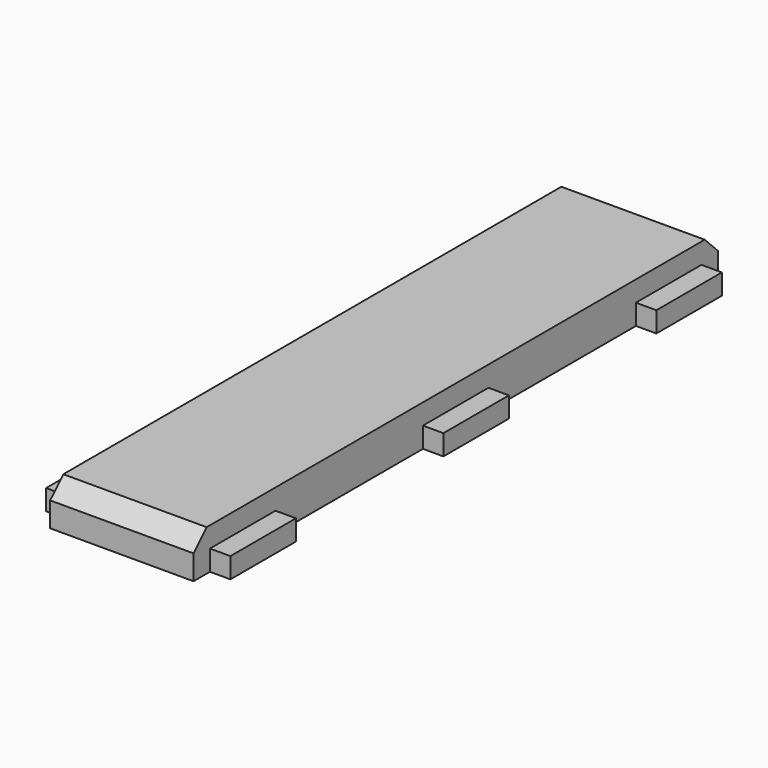
from build123d import *

# Parameters (mm, degrees)
F0_W     = 22.225
F0_H     = 101.6
F1_DEPTH = 6.35
F2_W     = 12.7
F2_H     = 3.175
F3_DEPTH = 3.175
F4_SIZE  = 2.54


# Not quite as in the source:
# - a pattern or mirror of a feature is missing from the dataset's text; its kind, count and spacing are read off the source's solid


with BuildPart() as f1:
    # F0 (on Top) → F1 (new body)
    with BuildSketch(Plane.XY):
        Rectangle(F0_W, F0_H)
    extrude(amount=F1_DEPTH)

    # F2 (on face) → F3 (join)
    with BuildSketch(Plane.YZ.offset(11.1125)):
        with Locations((-41.275, 1.5875)):
            Rectangle(F2_W, F2_H)
        with Locations((0, 1.5875)):
            Rectangle(F2_W, F2_H)
        with Locations((41.275, 1.5875)):
            Rectangle(F2_W, F2_H)
    f3 = extrude(amount=F3_DEPTH)

    # F3_copies: F3 across plane
    add(f3.mirror(Plane(origin=(0, 0, 0), x_dir=(0, 0, -1), z_dir=(-1, 0, 0))))

    # F4
    f4_edges = [f1.edges().sort_by_distance(p)[0] for p in [
        (0, 50.8, 6.35),
        (0, -50.8, 6.35),
    ]]
    chamfer(f4_edges, length=F4_SIZE)


solid = f1.part
